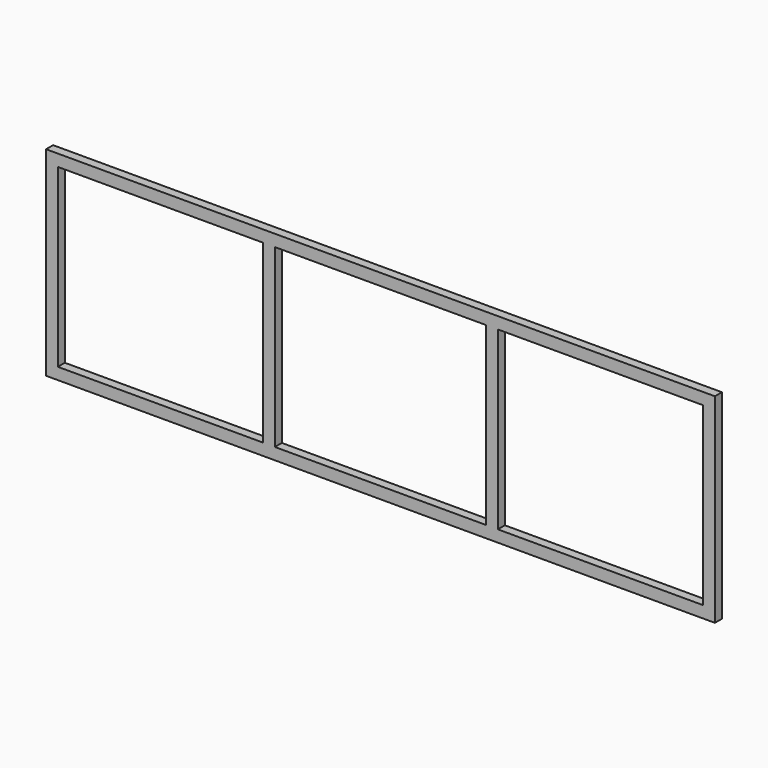
from build123d import *

# Parameters (mm, degrees)
F1_W     = 1447.8
F1_H     = 431.8
F1_W_2   = 25.4
F1_H_2   = 381
F2_DEPTH = 19.05


# Not quite as in the source:
# - a variable given as a bare number and used for a length is read in inches; the dataset says mm whatever the document's units were


with BuildPart() as f2:
    # F1 (on Front) → F2 (new body)
    with BuildSketch(Plane.XZ):
        Rectangle(F1_W, F1_H)
        Polygon((-698.5, -190.5), (-698.5, 190.5), (-254, 190.5), (-228.6, 190.5), (228.6, 190.5), (254, 190.5), (698.5, 190.5), (698.5, -190.5), (254, -190.5), (228.6, -190.5), (-228.6, -190.5), (-254, -190.5), align=None, mode=Mode.SUBTRACT)
        with Locations((-241.3, 0)):
            Rectangle(F1_W_2, F1_H_2)
        with Locations((241.3, 0)):
            Rectangle(F1_W_2, F1_H_2)
    extrude(amount=F2_DEPTH)


solid = f2.part
